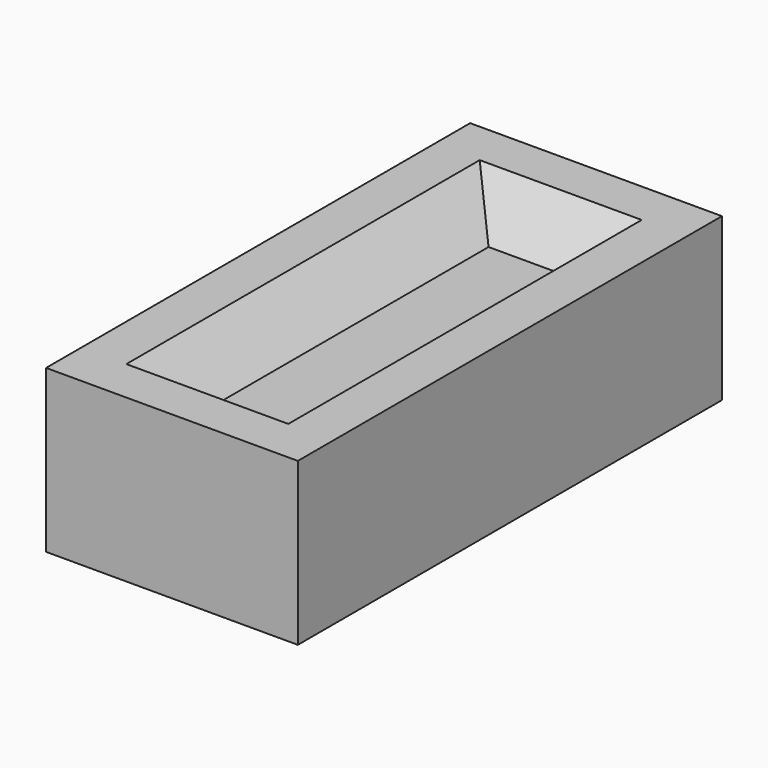
from build123d import *

# Parameters (mm, degrees)
F3_W     = 17.1
F3_H     = 36
F0_DEPTH = 5.5
F4_W     = 30
F4_H     = 3
F1_DEPTH = 5.5
F2_SIZE  = 2.99999


# Not quite as in the source:
# - a fillet or chamfer is up to 0.001 mm smaller than in the source, because OpenCascade refuses the exact size


with BuildPart() as f0:
    # F3 (on Top) → F0 (new body, symmetric)
    with BuildSketch(Plane.XY):
        Rectangle(F3_W, F3_H)
    extrude(amount=F0_DEPTH, both=True)

    # F4 (on Right) → F1 (cut, symmetric)
    with BuildSketch(Plane.YZ):
        with Locations((0, 4)):
            Rectangle(F4_W, F4_H)
    extrude(amount=F1_DEPTH, both=True, mode=Mode.SUBTRACT)

    # F2 (size 3 in the source; OpenCascade refuses exactly that, so slightly less here)
    f2_edges = [f0.edges().sort_by_distance(p)[0] for p in [
        (-5.5, 0, 2.5),
        (0, -15, 2.5),
        (0, 15, 2.5),
        (5.5, 0, 2.5),
    ]]
    chamfer(f2_edges, length=F2_SIZE)


solid = f0.part
